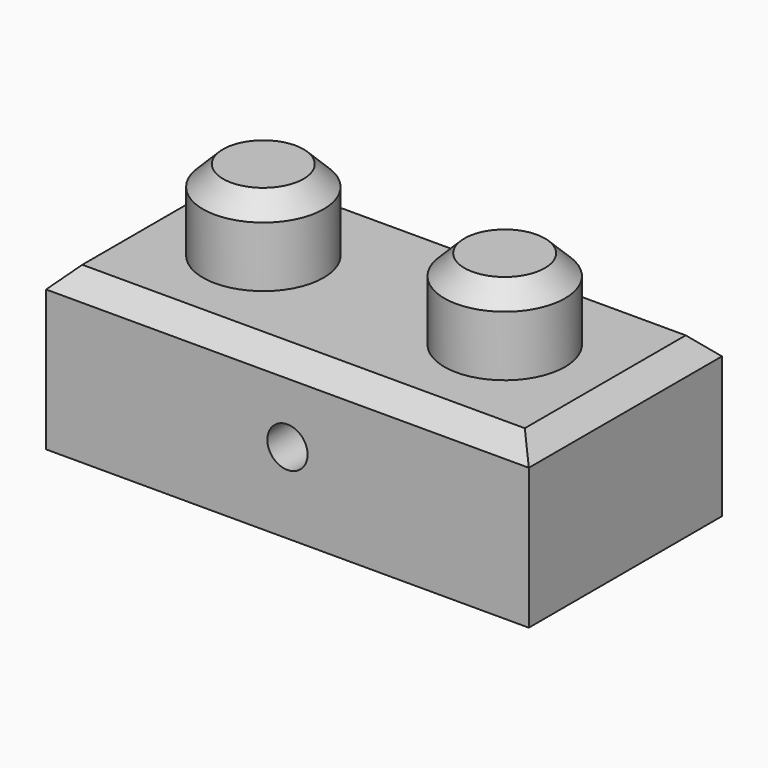
from build123d import *

# Parameters (mm, degrees)
F0_W     = 76.2
F0_H     = 38.1
F1_DEPTH = 25.4
F2_R     = 9.525
F3_DEPTH = 12.7
F4_SIZE  = 3.175
F5_T     = 7.9375
F6_R     = 3.175
F7_DEPTH = 7.9375
F8_R     = 3.175
F9_DEPTH = 7.9375


# Not quite as in the source:
# - a length typed as a fraction of an inch, garbled in the dataset ("3 / 203.2 mm" for 3/8 in), is restored
# - a shell that OpenCascade refuses in one call is made with other operations: the cavity is built on its own and cut out


with BuildPart() as f1:
    # F0 (on Top) → F1 (new body)
    with BuildSketch(Plane.XY):
        with Locations((69.7679412603, -31.8402817965)):
            Rectangle(F0_W, F0_H)
    extrude(amount=F1_DEPTH)

    # F2 (on face) → F3 (join)
    with BuildSketch(Plane.XY.offset(25.4)):
        with Locations((88.8179412603, -31.8402817965)):
            Circle(F2_R)
        with Locations((50.7179412603, -31.8402817965)):
            Circle(F2_R)
    extrude(amount=F3_DEPTH)

    # F4
    f4_edges = [f1.edges().sort_by_distance(p)[0] for p in [
        (41.192941, -31.840282, 38.1),
        (79.292941, -31.840282, 38.1),
        (69.767941, -50.890282, 25.4),
        (31.667941, -31.840282, 25.4),
        (107.867941, -31.840282, 25.4),
        (69.767941, -12.790282, 25.4),
    ]]
    chamfer(f4_edges, length=F4_SIZE)

    # F5: shell of thickness 7.9375, made by hand


with BuildPart() as f5_core1:
    # F5_t2: copy of F1
    add(f1.part)

    # the walls: a layer under each face that stays
    f5_faces = [f5_core1.faces().sort_by_distance(p)[0] for p in [
        (69.7679412603, -12.7902817965, 11.1125),
        (107.8679412603, -31.8402817965, 11.1125),
        (69.7679412603, -14.3777817965, 23.8125),
        (31.6679412603, -31.8402817965, 11.1125),
        (69.7679412603, -50.8902817965, 11.1125),
        (106.2804412603, -31.8402817965, 23.8125),
        (69.7679412603, -31.8402817965, 25.4),
        (33.2554412603, -31.8402817965, 23.8125),
        (69.7679412603, -49.3027817965, 23.8125),
        (41.1929412603, -31.8402817965, 30.1625),
        (79.2929412603, -31.8402817965, 30.1625),
        (42.7804412603, -31.8402817965, 36.5125),
        (80.8804412603, -31.8402817965, 36.5125),
        (50.7179412603, -31.8402817965, 38.1),
        (88.8179412603, -31.8402817965, 38.1),
    ]]
    thicken(f5_faces, amount=-F5_T, mode=Mode.SUBTRACT)

    # F5_s3 → F5_t4 (revolve, cut)
    with BuildSketch(Plane.XZ.offset(31.8402817965)):
        Polygon((60.3223162603, 25.479375), (60.2429412603, 17.4625), (52.3054412603, 17.4625), (52.3054412603, 25.4), align=None)
    revolve(axis=Axis((50.7179412603, -31.8402817965, 25.4), (0, 0, 1)), mode=Mode.SUBTRACT)

    # F5_s5 → F5_t6 (revolve, cut)
    with BuildSketch(Plane.XZ.offset(31.8402817965)):
        Polygon((98.4223162603, 25.479375), (98.3429412603, 17.4625), (90.4054412603, 17.4625), (90.4054412603, 25.4), align=None)
    revolve(axis=Axis((88.8179412603, -31.8402817965, 25.4), (0, 0, 1)), mode=Mode.SUBTRACT)


with BuildPart() as f1_1:
    add(f1.part)

    # what is left inside the walls is the cavity
    f5_cavity = [f5_core1.part.solids().sort_by_distance(p)[0] for p in [
        (69.767941, -35.544448, 0.079375),
    ]]
    add(f5_cavity, mode=Mode.SUBTRACT)

    # F6 (on face) → F7 (cut)
    with BuildSketch(Plane(origin=(0, -12.7902817965, 0), x_dir=(-1, 0, 0), z_dir=(0, 1, 0))):
        with Locations((-69.7679412603, 12.7)):
            Circle(F6_R)
    extrude(amount=-F7_DEPTH, mode=Mode.SUBTRACT)

    # F8 (on face) → F9 (cut)
    with BuildSketch(Plane.XZ.offset(50.8902817965)):
        with Locations((69.7679412603, 12.7)):
            Circle(F8_R)
    extrude(amount=-F9_DEPTH, mode=Mode.SUBTRACT)


solid = f1_1.part
